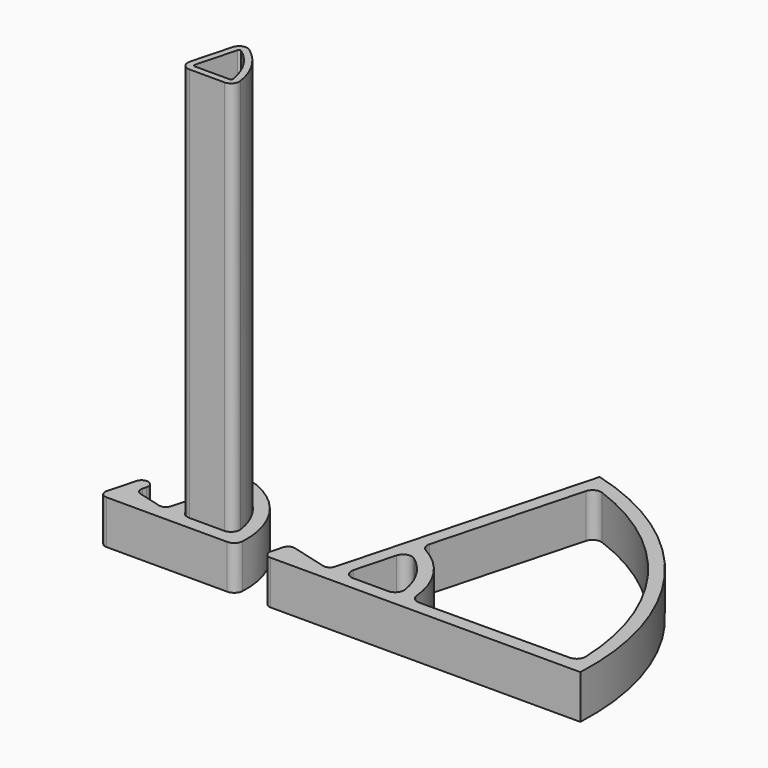
from build123d import *

# Parameters (mm, degrees)
F1_DEPTH     = 100
F2_DEPTH     = 10
F3_DEPTH     = 10
F4_TEXT_SIZE = 8.3333333333
F5_DEPTH     = 1


# Not quite as in the source:
# - Text() gives the source's letters only with a copy of the font that has no kerning and outlines rounded to 1/6400 em; it was checked with that copy


with BuildPart() as f1:
    # F0 (on Top) → F1 (new body)
    with BuildSketch(Plane.XY):
        with BuildLine():
            Line((6.3328192079, 14.656922793), (3.877020217, 5.4917561857))
            ThreePointArc((3.877020217, 5.4917561857), (4.2049079404, 3.8433532849), (5.7122792869, 3.1))
            Line((5.7122792869, 3.1), (13.688624771, 3.1))
            ThreePointArc((13.688624771, 3.1), (15.1259667745, 3.7574027341), (15.5686639748, 5.2746863524))
            ThreePointArc((15.5686639748, 5.2746863524), (13.4778255299, 11.1182334869), (9.2899080919, 15.6986260519))
            ThreePointArc((9.2899080919, 15.6986260519), (7.5367845699, 15.957223597), (6.3328192079, 14.656922793))
        make_face()
        with BuildLine():
            ThreePointArc((14.0844224982, 5.0578287058), (13.9912230875, 4.7384005756), (13.688624771, 4.6))
            Line((13.688624771, 4.6), (5.7122792869, 4.6))
            ThreePointArc((5.7122792869, 4.6), (5.3949379508, 4.7564954284), (5.3259089564, 5.103527618))
            Line((5.3259089564, 5.103527618), (7.7817079473, 14.2686942254))
            ThreePointArc((7.7817079473, 14.2686942254), (8.0351743393, 14.5424417631), (8.4042529755, 14.4880001746))
            ThreePointArc((8.4042529755, 14.4880001746), (12.1929145254, 10.344280187), (14.0844224982, 5.0578287058))
        make_face(mode=Mode.SUBTRACT)
    extrude(amount=F1_DEPTH)


with BuildPart() as f2:
    # F0 (on Top) → F2 (new body)
    with BuildSketch(Plane.XY):
        with BuildLine():
            ThreePointArc((16.8042318441, 0), (18.1757975704, 0.5443876002), (18.8006999225, 1.8811925414))
            ThreePointArc((18.8006999225, 1.8811925414), (15.90871964, 13.0812046463), (7.015783132, 20.478467746))
            ThreePointArc((7.015783132, 20.478467746), (5.3763483707, 20.4112666935), (4.3389173509, 19.1400471226))
            Line((4.3389173509, 19.1400471226), (0.389098349, 4.4473808049))
            ThreePointArc((0.389098349, 4.4473808049), (-0.3100044739, 3.537452863), (-1.4476997505, 3.387909979))
            Line((-1.4476997505, 3.387909979), (-6.761480784, 4.8117333157))
            ThreePointArc((-6.761480784, 4.8117333157), (-7.672290322, 5.5106220552), (-7.8221409558, 6.6488506228))
            Line((-7.8221409558, 6.6488506228), (-7.5974400228, 7.4874459213))
            ThreePointArc((-7.5974400228, 7.4874459213), (-8.6581001946, 9.3245632284), (-10.4952175017, 8.2639030566))
            Line((-10.4952175017, 8.2639030566), (-12.2035743322, 1.8882285677))
            ThreePointArc((-12.2035743322, 1.8882285677), (-11.9447156032, 0.5868578565), (-10.7546855927, 0))
            Line((-10.7546855927, 0), (16.8042318441, 0))
        make_face()
        with BuildLine():
            ThreePointArc((9.3489517664, 15.7793344437), (13.5634862635, 11.1698303736), (15.6676134066, 5.2891435288))
            ThreePointArc((15.6676134066, 5.2891435288), (15.2016163536, 3.692002878), (13.688624771, 3))
            Line((13.688624771, 3), (5.7122792869, 3))
            ThreePointArc((5.7122792869, 3), (4.1255726063, 3.782477142), (3.7804276343, 5.5176380902))
            Line((3.7804276343, 5.5176380902), (6.2362266253, 14.6828046975))
            ThreePointArc((6.2362266253, 14.6828046975), (7.5035585853, 16.051542386), (9.3489517664, 15.7793344437))
        make_face(mode=Mode.SUBTRACT)
    extrude(amount=F2_DEPTH)


with BuildPart() as f3:
    # F0 (on Top) → F3 (new body)
    with BuildSketch(Plane.XY):
        with BuildLine():
            Line((35.9233482484, 3.4516239499), (30.6095672732, 4.875447271))
            Line((30.6095672732, 4.875447271), (27.7117897944, 5.6519044063))
            ThreePointArc((27.7117897944, 5.6519044063), (26.5735612267, 5.5020537725), (25.8746724873, 4.5912442345))
            Line((25.8746724873, 4.5912442345), (25.1674737251, 1.9519425229))
            ThreePointArc((25.1674737251, 1.9519425229), (25.4263324541, 0.6505718117), (26.6163624645, 0.0637139552))
            Line((26.6163624645, 0.0637139552), (54.1752799014, 0.0637139552))
            Line((54.1752799014, 0.0637139552), (97.2960011236, 0.0637139552))
            ThreePointArc((97.2960011236, 0.0637139552), (85.8852841818, 38.3676640635), (52.9477622645, 61.0064958569))
            Line((52.9477622645, 61.0064958569), (41.7103910183, 19.2053468724))
            Line((41.7103910183, 19.2053468724), (37.7601463636, 4.5110948342))
            ThreePointArc((37.7601463636, 4.5110948342), (37.0610435511, 3.601166849), (35.9233482484, 3.4516239499))
        make_face()
        with BuildLine():
            ThreePointArc((46.7199998236, 15.843048399), (50.9345343208, 11.2335443289), (53.0386614639, 5.3528574841))
            ThreePointArc((53.0386614639, 5.3528574841), (52.5726644108, 3.7557168332), (51.0596728283, 3.0637139552))
            Line((51.0596728283, 3.0637139552), (43.0833273442, 3.0637139552))
            ThreePointArc((43.0833273442, 3.0637139552), (41.4966206636, 3.8461910972), (41.1514756916, 5.5813520455))
            Line((41.1514756916, 5.5813520455), (43.6072746825, 14.7465186528))
            ThreePointArc((43.6072746825, 14.7465186528), (44.8746066425, 16.1152563412), (46.7199998236, 15.843048399))
        make_face(mode=Mode.SUBTRACT)
        with BuildLine():
            ThreePointArc((58.119245281, 3.0637412904), (56.7680426065, 3.5796654804), (56.1180254889, 4.87171973))
            ThreePointArc((56.1180254889, 4.87171973), (53.1105709635, 13.4070918554), (46.4691728521, 19.5543832237))
            ThreePointArc((46.4691728521, 19.5543832237), (45.5950811018, 20.5222549341), (45.5034615986, 21.8231845642))
            Line((45.5034615986, 21.8231845642), (54.4449284676, 55.1931932135))
            ThreePointArc((54.4449284676, 55.1931932135), (55.4566270676, 56.4513136541), (57.0678976497, 56.5523493476))
            ThreePointArc((57.0678976497, 56.5523493476), (83.4690636192, 36.5894199322), (94.3263005988, 5.3218565389))
            ThreePointArc((94.3263005988, 5.3218565389), (93.7734433566, 3.8604803287), (92.3383272523, 3.2426508009))
            Line((92.3383272523, 3.2426508009), (58.119245281, 3.0637412904))
        make_face(mode=Mode.SUBTRACT)
    extrude(amount=F3_DEPTH)

    # F4 (on face) → F5 (cut)
    with BuildSketch(Plane(origin=(34.0841958797, -9.1628285833, 0), x_dir=(-0.2596119035, -0.9657130317, 0), z_dir=(-0.9657130317, 0.2596119035, 0))):
        with Locations((-54.2759073931, 2.434563267)):
            Text('Plexy', F4_TEXT_SIZE, font='Arimo', font_style=FontStyle.BOLD, text_align=(TextAlign.LEFT, TextAlign.BOTTOM))
    extrude(amount=-F5_DEPTH, mode=Mode.SUBTRACT)


solid = Compound([f1.part, f2.part, f3.part])
